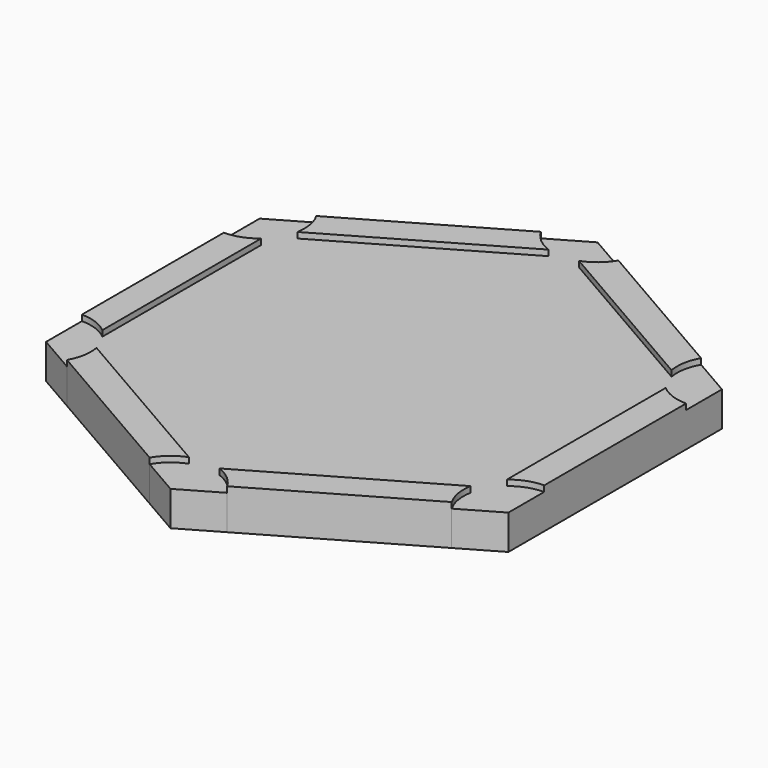
from build123d import *

# Parameters (mm, degrees)
F1_DEPTH        = 6
F2_DEPTH        = 7
F2_COPIES_COUNT = 6
F4_DEPTH        = 5
F5_START        = 1
F5_DEPTH        = 4


# Not quite as in the source:
# - a pattern or mirror of a feature is missing from the dataset's text; its kind, count and spacing are read off the source's solid


with BuildPart() as f1:
    # F0 (on Top) → F1 (new body)
    with BuildSketch(Plane.XY):
        with BuildLine():
            ThreePointArc((-33.2883031207, -26.9690107676), (-32.3656613578, -24.4279423614), (-32.3719521258, -21.7245635692))
            Line((-32.3719521258, -21.7245635692), (-35, -20.2072594216))
            Line((-35, -20.2072594216), (-35, -17.1726511264))
            ThreePointArc((-35, -17.1726511264), (-37.3380493261, -15.8155137655), (-40, -15.3440107676))
            Line((-40, -15.3440107676), (-40, -23.0940107676))
            Line((-40, -23.0940107676), (-33.2883031207, -26.9690107676))
        make_face()
        with BuildLine():
            Line((0, -46.1880215352), (6.7116968793, -42.3130215352))
            ThreePointArc((6.7116968793, -42.3130215352), (4.9723879682, -40.2434561269), (2.6280478742, -38.8972146957))
            Line((2.6280478742, -38.8972146957), (0, -40.4145188433))
            Line((0, -40.4145188433), (-2.6280478742, -38.8972146957))
            ThreePointArc((-2.6280478742, -38.8972146957), (-4.9723879682, -40.2434561269), (-6.7116968793, -42.3130215352))
            Line((-6.7116968793, -42.3130215352), (0, -46.1880215352))
        make_face()
        with BuildLine():
            Line((40, -23.0940107676), (40, -15.3440107676))
            ThreePointArc((40, -15.3440107676), (37.3380493261, -15.8155137655), (35, -17.1726511264))
            Line((35, -17.1726511264), (35, -20.2072594216))
            Line((35, -20.2072594216), (32.3719521258, -21.7245635692))
            ThreePointArc((32.3719521258, -21.7245635692), (32.3656613578, -24.4279423614), (33.2883031207, -26.9690107676))
            Line((33.2883031207, -26.9690107676), (40, -23.0940107676))
        make_face()
        with BuildLine():
            Line((40, 15.3440107676), (40, 23.0940107676))
            Line((40, 23.0940107676), (33.2883031207, 26.9690107676))
            ThreePointArc((33.2883031207, 26.9690107676), (32.3656613578, 24.4279423614), (32.3719521258, 21.7245635692))
            Line((32.3719521258, 21.7245635692), (35, 20.2072594216))
            Line((35, 20.2072594216), (35, 17.1726511264))
            ThreePointArc((35, 17.1726511264), (37.3380493261, 15.8155137655), (40, 15.3440107676))
        make_face()
        with BuildLine():
            ThreePointArc((2.6280478742, 38.8972146957), (4.9723879682, 40.2434561269), (6.7116968793, 42.3130215352))
            Line((6.7116968793, 42.3130215352), (0, 46.1880215352))
            Line((0, 46.1880215352), (-6.7116968793, 42.3130215352))
            ThreePointArc((-6.7116968793, 42.3130215352), (-4.9723879682, 40.2434561269), (-2.6280478742, 38.8972146957))
            Line((-2.6280478742, 38.8972146957), (0, 40.4145188433))
            Line((0, 40.4145188433), (2.6280478742, 38.8972146957))
        make_face()
        with BuildLine():
            ThreePointArc((-32.3719521258, 21.7245635692), (-32.3656613578, 24.4279423614), (-33.2883031207, 26.9690107676))
            Line((-33.2883031207, 26.9690107676), (-40, 23.0940107676))
            Line((-40, 23.0940107676), (-40, 15.3440107676))
            ThreePointArc((-40, 15.3440107676), (-37.3380493261, 15.8155137655), (-35, 17.1726511264))
            Line((-35, 17.1726511264), (-35, 20.2072594216))
            Line((-35, 20.2072594216), (-32.3719521258, 21.7245635692))
        make_face()
        with BuildLine():
            ThreePointArc((-35, 17.1726511264), (-33.2883031207, 19.2190107676), (-32.3719521258, 21.7245635692))
            Line((-32.3719521258, 21.7245635692), (-35, 20.2072594216))
            Line((-35, 20.2072594216), (-35, 17.1726511264))
        make_face()
        with BuildLine():
            ThreePointArc((-2.6280478742, 38.8972146957), (0, 38.4380215352), (2.6280478742, 38.8972146957))
            Line((2.6280478742, 38.8972146957), (0, 40.4145188433))
            Line((0, 40.4145188433), (-2.6280478742, 38.8972146957))
        make_face()
        with BuildLine():
            Line((-35, -20.2072594216), (-32.3719521258, -21.7245635692))
            ThreePointArc((-32.3719521258, -21.7245635692), (-33.2883031207, -19.2190107676), (-35, -17.1726511264))
            Line((-35, -17.1726511264), (-35, -20.2072594216))
        make_face()
        with BuildLine():
            Line((0, -40.4145188433), (2.6280478742, -38.8972146957))
            ThreePointArc((2.6280478742, -38.8972146957), (0, -38.4380215352), (-2.6280478742, -38.8972146957))
            Line((-2.6280478742, -38.8972146957), (0, -40.4145188433))
        make_face()
        with BuildLine():
            Line((35, -20.2072594216), (35, -17.1726511264))
            ThreePointArc((35, -17.1726511264), (33.2883031207, -19.2190107676), (32.3719521258, -21.7245635692))
            Line((32.3719521258, -21.7245635692), (35, -20.2072594216))
        make_face()
        with BuildLine():
            ThreePointArc((32.3719521258, 21.7245635692), (33.2883031207, 19.2190107676), (35, 17.1726511264))
            Line((35, 17.1726511264), (35, 20.2072594216))
            Line((35, 20.2072594216), (32.3719521258, 21.7245635692))
        make_face()
        with BuildLine():
            Line((35, -17.1726511264), (35, 17.1726511264))
            ThreePointArc((35, 17.1726511264), (33.2883031207, 19.2190107676), (32.3719521258, 21.7245635692))
            Line((32.3719521258, 21.7245635692), (2.6280478742, 38.8972146957))
            ThreePointArc((2.6280478742, 38.8972146957), (0, 38.4380215352), (-2.6280478742, 38.8972146957))
            Line((-2.6280478742, 38.8972146957), (-32.3719521258, 21.7245635692))
            ThreePointArc((-32.3719521258, 21.7245635692), (-33.2883031207, 19.2190107676), (-35, 17.1726511264))
            Line((-35, 17.1726511264), (-35, -17.1726511264))
            ThreePointArc((-35, -17.1726511264), (-33.2883031207, -19.2190107676), (-32.3719521258, -21.7245635692))
            Line((-32.3719521258, -21.7245635692), (-2.6280478742, -38.8972146957))
            ThreePointArc((-2.6280478742, -38.8972146957), (0, -38.4380215352), (2.6280478742, -38.8972146957))
            Line((2.6280478742, -38.8972146957), (32.3719521258, -21.7245635692))
            ThreePointArc((32.3719521258, -21.7245635692), (33.2883031207, -19.2190107676), (35, -17.1726511264))
        make_face()
    extrude(amount=F1_DEPTH)

    # F0 (on Top) → F2 (join)
    with BuildSketch(Plane.XY):
        with BuildLine():
            Line((40, -15.3440107676), (40, 15.3440107676))
            ThreePointArc((40, 15.3440107676), (37.3380493261, 15.8155137655), (35, 17.1726511264))
            Line((35, 17.1726511264), (35, -17.1726511264))
            ThreePointArc((35, -17.1726511264), (37.3380493261, -15.8155137655), (40, -15.3440107676))
        make_face()
    f2 = extrude(amount=F2_DEPTH)

    # F2_copies: F2 ×6 about axis
    f2_copies_axis = Axis((0, 0, 0), (0, 0, 1))
    for i in range(1, F2_COPIES_COUNT):
        add(f2.rotate(f2_copies_axis, i * 360 / F2_COPIES_COUNT))

    # F3 (on face) → F4 (cut)
    with BuildSketch(Plane.XY):
        with BuildLine():
            Line((-36, -12.1346096908), (-36, -7.4346096908))
            ThreePointArc((-36, -7.4346096908), (-38.35, -9.7846096908), (-36, -12.1346096908))
        make_face()
        with BuildLine():
            ThreePointArc((-33.65, -9.7846096908), (-34.3382990642, -8.122908755), (-36, -7.4346096908))
            Line((-36, -7.4346096908), (-36, -12.1346096908))
            ThreePointArc((-36, -12.1346096908), (-34.3382990642, -11.4463106266), (-33.65, -9.7846096908))
        make_face()
        with BuildLine():
            ThreePointArc((-33.65, 9.7846096908), (-34.3382990642, 11.4463106266), (-36, 12.1346096908))
            Line((-36, 12.1346096908), (-36, 7.4346096908))
            ThreePointArc((-36, 7.4346096908), (-34.3382990642, 8.122908755), (-33.65, 9.7846096908))
        make_face()
        with BuildLine():
            Line((-36, 7.4346096908), (-36, 12.1346096908))
            ThreePointArc((-36, 12.1346096908), (-38.35, 9.7846096908), (-36, 7.4346096908))
        make_face()
        with BuildLine():
            ThreePointArc((-24.1237205584, 26.2846096908), (-24.2037948666, 26.8928344468), (-24.4385608595, 27.4596096908))
            Line((-24.4385608595, 27.4596096908), (-28.5088802573, 25.1096096908))
            ThreePointArc((-28.5088802573, 25.1096096908), (-25.8654958024, 24.014683999), (-24.1237205584, 26.2846096908))
        make_face()
        with BuildLine():
            Line((-28.5088802573, 25.1096096908), (-24.4385608595, 27.4596096908))
            ThreePointArc((-24.4385608595, 27.4596096908), (-27.6487205584, 28.3197693897), (-28.5088802573, 25.1096096908))
        make_face()
        with BuildLine():
            ThreePointArc((-7.1762794416, 36.0692193817), (-7.2563537498, 36.6774441376), (-7.4911197427, 37.2442193817))
            Line((-7.4911197427, 37.2442193817), (-11.5614391405, 34.8942193817))
            ThreePointArc((-11.5614391405, 34.8942193817), (-8.9180546856, 33.7992936899), (-7.1762794416, 36.0692193817))
        make_face()
        with BuildLine():
            Line((-11.5614391405, 34.8942193817), (-7.4911197427, 37.2442193817))
            ThreePointArc((-7.4911197427, 37.2442193817), (-10.7012794416, 38.1043790805), (-11.5614391405, 34.8942193817))
        make_face()
        with BuildLine():
            ThreePointArc((7.4911197427, 37.2442193817), (8.3512794416, 34.0340596828), (11.5614391405, 34.8942193817))
            Line((11.5614391405, 34.8942193817), (7.4911197427, 37.2442193817))
        make_face()
        with BuildLine():
            Line((7.4911197427, 37.2442193817), (11.5614391405, 34.8942193817))
            ThreePointArc((11.5614391405, 34.8942193817), (11.7962051334, 35.4609946257), (11.8762794416, 36.0692193817))
            ThreePointArc((11.8762794416, 36.0692193817), (10.1345041976, 38.3391450734), (7.4911197427, 37.2442193817))
        make_face()
        with BuildLine():
            ThreePointArc((24.4385608595, 27.4596096908), (25.2987205584, 24.2494499919), (28.5088802573, 25.1096096908))
            Line((28.5088802573, 25.1096096908), (24.4385608595, 27.4596096908))
        make_face()
        with BuildLine():
            Line((24.4385608595, 27.4596096908), (28.5088802573, 25.1096096908))
            ThreePointArc((28.5088802573, 25.1096096908), (28.7436462502, 25.6763849348), (28.8237205584, 26.2846096908))
            ThreePointArc((28.8237205584, 26.2846096908), (27.0819453144, 28.5545353826), (24.4385608595, 27.4596096908))
        make_face()
        with BuildLine():
            Line((36, 7.4346096908), (36, 12.1346096908))
            ThreePointArc((36, 12.1346096908), (33.65, 9.7846096908), (36, 7.4346096908))
        make_face()
        with BuildLine():
            ThreePointArc((38.35, 9.7846096908), (37.6617009358, 11.4463106266), (36, 12.1346096908))
            Line((36, 12.1346096908), (36, 7.4346096908))
            ThreePointArc((36, 7.4346096908), (37.6617009358, 8.122908755), (38.35, 9.7846096908))
        make_face()
        with BuildLine():
            Line((36, -12.1346096908), (36, -7.4346096908))
            ThreePointArc((36, -7.4346096908), (33.65, -9.7846096908), (36, -12.1346096908))
        make_face()
        with BuildLine():
            ThreePointArc((38.35, -9.7846096908), (37.6617009358, -8.122908755), (36, -7.4346096908))
            Line((36, -7.4346096908), (36, -12.1346096908))
            ThreePointArc((36, -12.1346096908), (37.6617009358, -11.4463106266), (38.35, -9.7846096908))
        make_face()
        with BuildLine():
            ThreePointArc((28.8237205584, -26.2846096908), (28.7436462502, -25.6763849348), (28.5088802573, -25.1096096908))
            Line((28.5088802573, -25.1096096908), (24.4385608595, -27.4596096908))
            ThreePointArc((24.4385608595, -27.4596096908), (27.0819453144, -28.5545353826), (28.8237205584, -26.2846096908))
        make_face()
        with BuildLine():
            Line((24.4385608595, -27.4596096908), (28.5088802573, -25.1096096908))
            ThreePointArc((28.5088802573, -25.1096096908), (25.2987205584, -24.2494499919), (24.4385608595, -27.4596096908))
        make_face()
        with BuildLine():
            ThreePointArc((11.8762794416, -36.0692193817), (11.7962051334, -35.4609946257), (11.5614391405, -34.8942193817))
            Line((11.5614391405, -34.8942193817), (7.4911197427, -37.2442193817))
            ThreePointArc((7.4911197427, -37.2442193817), (10.1345041976, -38.3391450734), (11.8762794416, -36.0692193817))
        make_face()
        with BuildLine():
            Line((7.4911197427, -37.2442193817), (11.5614391405, -34.8942193817))
            ThreePointArc((11.5614391405, -34.8942193817), (8.3512794416, -34.0340596828), (7.4911197427, -37.2442193817))
        make_face()
        with BuildLine():
            Line((-9.5262794416, -36.0692193817), (-7.4911197427, -37.2442193817))
            ThreePointArc((-7.4911197427, -37.2442193817), (-7.2563537498, -36.6774441376), (-7.1762794416, -36.0692193817))
            ThreePointArc((-7.1762794416, -36.0692193817), (-8.9180546856, -33.7992936899), (-11.5614391405, -34.8942193817))
            Line((-11.5614391405, -34.8942193817), (-9.5262794416, -36.0692193817))
        make_face()
        with BuildLine():
            ThreePointArc((-11.5614391405, -34.8942193817), (-10.7012794416, -38.1043790805), (-7.4911197427, -37.2442193817))
            Line((-7.4911197427, -37.2442193817), (-9.5262794416, -36.0692193817))
            Line((-9.5262794416, -36.0692193817), (-11.5614391405, -34.8942193817))
        make_face()
        with BuildLine():
            Line((-26.4737205584, -26.2846096908), (-24.4385608595, -27.4596096908))
            ThreePointArc((-24.4385608595, -27.4596096908), (-24.2037948666, -26.8928344468), (-24.1237205584, -26.2846096908))
            ThreePointArc((-24.1237205584, -26.2846096908), (-25.8654958024, -24.014683999), (-28.5088802573, -25.1096096908))
            Line((-28.5088802573, -25.1096096908), (-26.4737205584, -26.2846096908))
        make_face()
        with BuildLine():
            ThreePointArc((-28.5088802573, -25.1096096908), (-27.6487205584, -28.3197693897), (-24.4385608595, -27.4596096908))
            Line((-24.4385608595, -27.4596096908), (-26.4737205584, -26.2846096908))
            Line((-26.4737205584, -26.2846096908), (-28.5088802573, -25.1096096908))
        make_face()
    extrude(amount=F4_DEPTH, mode=Mode.SUBTRACT)

    # F3 (on face) → F5 (cut)
    with BuildSketch(Plane.XY.offset(F5_START)):
        with BuildLine():
            ThreePointArc((39.5, 11.7211013639), (38.0315060063, 13.2303292595), (36, 13.7846096908))
            Line((36, 13.7846096908), (36, 12.1346096908))
            ThreePointArc((36, 12.1346096908), (37.6617009358, 11.4463106266), (38.35, 9.7846096908))
            ThreePointArc((38.35, 9.7846096908), (37.6617009358, 8.122908755), (36, 7.4346096908))
            Line((36, 7.4346096908), (36, 5.7846096908))
            ThreePointArc((36, 5.7846096908), (38.0315060063, 6.3388901221), (39.5, 7.8481180177))
            Line((39.5, 7.8481180177), (39.5, 11.7211013639))
        make_face()
        with BuildLine():
            Line((36, 12.1346096908), (36, 13.7846096908))
            ThreePointArc((36, 13.7846096908), (32, 9.7846096908), (36, 5.7846096908))
            Line((36, 5.7846096908), (36, 7.4346096908))
            ThreePointArc((36, 7.4346096908), (33.65, 9.7846096908), (36, 12.1346096908))
        make_face()
        with BuildLine():
            ThreePointArc((23.0096189432, 28.2846096908), (24.4737205584, 22.8205080757), (29.9378221735, 24.2846096908))
            Line((29.9378221735, 24.2846096908), (28.5088802573, 25.1096096908))
            ThreePointArc((28.5088802573, 25.1096096908), (25.2987205584, 24.2494499919), (24.4385608595, 27.4596096908))
            Line((24.4385608595, 27.4596096908), (23.0096189432, 28.2846096908))
        make_face()
        with BuildLine():
            Line((28.5088802573, 25.1096096908), (29.9378221735, 24.2846096908))
            ThreePointArc((29.9378221735, 24.2846096908), (30.4735542424, 26.3210857159), (29.9007715415, 28.3474527675))
            Line((29.9007715415, 28.3474527675), (26.5466695752, 30.2839444406))
            ThreePointArc((26.5466695752, 30.2839444406), (24.5053928807, 29.7668052846), (23.0096189432, 28.2846096908))
            Line((23.0096189432, 28.2846096908), (24.4385608595, 27.4596096908))
            ThreePointArc((24.4385608595, 27.4596096908), (27.0819453144, 28.5545353826), (28.8237205584, 26.2846096908))
            ThreePointArc((28.8237205584, 26.2846096908), (28.7436462502, 25.6763849348), (28.5088802573, 25.1096096908))
        make_face()
        with BuildLine():
            ThreePointArc((39.5, -7.8481180177), (38.0315060063, -6.3388901221), (36, -5.7846096908))
            Line((36, -5.7846096908), (36, -7.4346096908))
            ThreePointArc((36, -7.4346096908), (37.6617009358, -8.122908755), (38.35, -9.7846096908))
            ThreePointArc((38.35, -9.7846096908), (37.6617009358, -11.4463106266), (36, -12.1346096908))
            Line((36, -12.1346096908), (36, -13.7846096908))
            ThreePointArc((36, -13.7846096908), (38.0315060063, -13.2303292595), (39.5, -11.7211013639))
            Line((39.5, -11.7211013639), (39.5, -7.8481180177))
        make_face()
        with BuildLine():
            Line((36, -7.4346096908), (36, -5.7846096908))
            ThreePointArc((36, -5.7846096908), (32, -9.7846096908), (36, -13.7846096908))
            Line((36, -13.7846096908), (36, -12.1346096908))
            ThreePointArc((36, -12.1346096908), (33.65, -9.7846096908), (36, -7.4346096908))
        make_face()
        with BuildLine():
            ThreePointArc((6.0621778265, 38.0692193817), (7.5262794416, 32.6051177665), (12.9903810568, 34.0692193817))
            Line((12.9903810568, 34.0692193817), (11.5614391405, 34.8942193817))
            ThreePointArc((11.5614391405, 34.8942193817), (8.3512794416, 34.0340596828), (7.4911197427, 37.2442193817))
            Line((7.4911197427, 37.2442193817), (6.0621778265, 38.0692193817))
        make_face()
        with BuildLine():
            Line((11.5614391405, 34.8942193817), (12.9903810568, 34.0692193817))
            ThreePointArc((12.9903810568, 34.0692193817), (13.5261131256, 36.1056954067), (12.9533304248, 38.1320624583))
            Line((12.9533304248, 38.1320624583), (9.5992284585, 40.0685541315))
            ThreePointArc((9.5992284585, 40.0685541315), (7.557951764, 39.5514149754), (6.0621778265, 38.0692193817))
            Line((6.0621778265, 38.0692193817), (7.4911197427, 37.2442193817))
            ThreePointArc((7.4911197427, 37.2442193817), (10.1345041976, 38.3391450734), (11.8762794416, 36.0692193817))
            ThreePointArc((11.8762794416, 36.0692193817), (11.7962051334, 35.4609946257), (11.5614391405, 34.8942193817))
        make_face()
        with BuildLine():
            ThreePointArc((29.9007715415, -28.3474527675), (30.4735542424, -26.3210857159), (29.9378221735, -24.2846096908))
            Line((29.9378221735, -24.2846096908), (28.5088802573, -25.1096096908))
            ThreePointArc((28.5088802573, -25.1096096908), (28.7436462502, -25.6763849348), (28.8237205584, -26.2846096908))
            ThreePointArc((28.8237205584, -26.2846096908), (27.0819453144, -28.5545353826), (24.4385608595, -27.4596096908))
            Line((24.4385608595, -27.4596096908), (23.0096189432, -28.2846096908))
            ThreePointArc((23.0096189432, -28.2846096908), (24.5053928807, -29.7668052846), (26.5466695752, -30.2839444406))
            Line((26.5466695752, -30.2839444406), (29.9007715415, -28.3474527675))
        make_face()
        with BuildLine():
            Line((28.5088802573, -25.1096096908), (29.9378221735, -24.2846096908))
            ThreePointArc((29.9378221735, -24.2846096908), (24.4737205584, -22.8205080757), (23.0096189432, -28.2846096908))
            Line((23.0096189432, -28.2846096908), (24.4385608595, -27.4596096908))
            ThreePointArc((24.4385608595, -27.4596096908), (25.2987205584, -24.2494499919), (28.5088802573, -25.1096096908))
        make_face()
        with BuildLine():
            ThreePointArc((-12.9903810568, 34.0692193817), (-7.5262794416, 32.6051177665), (-6.0621778265, 38.0692193817))
            Line((-6.0621778265, 38.0692193817), (-7.4911197427, 37.2442193817))
            ThreePointArc((-7.4911197427, 37.2442193817), (-7.2563537498, 36.6774441376), (-7.1762794416, 36.0692193817))
            ThreePointArc((-7.1762794416, 36.0692193817), (-8.9180546856, 33.7992936899), (-11.5614391405, 34.8942193817))
            Line((-11.5614391405, 34.8942193817), (-12.9903810568, 34.0692193817))
        make_face()
        with BuildLine():
            Line((-7.4911197427, 37.2442193817), (-6.0621778265, 38.0692193817))
            ThreePointArc((-6.0621778265, 38.0692193817), (-7.557951764, 39.5514149754), (-9.5992284585, 40.0685541315))
            Line((-9.5992284585, 40.0685541315), (-12.9533304248, 38.1320624583))
            ThreePointArc((-12.9533304248, 38.1320624583), (-13.5261131256, 36.1056954067), (-12.9903810568, 34.0692193817))
            Line((-12.9903810568, 34.0692193817), (-11.5614391405, 34.8942193817))
            ThreePointArc((-11.5614391405, 34.8942193817), (-10.7012794416, 38.1043790805), (-7.4911197427, 37.2442193817))
        make_face()
        with BuildLine():
            ThreePointArc((12.9533304248, -38.1320624583), (13.5261131256, -36.1056954067), (12.9903810568, -34.0692193817))
            Line((12.9903810568, -34.0692193817), (11.5614391405, -34.8942193817))
            ThreePointArc((11.5614391405, -34.8942193817), (11.7962051334, -35.4609946257), (11.8762794416, -36.0692193817))
            ThreePointArc((11.8762794416, -36.0692193817), (10.1345041976, -38.3391450734), (7.4911197427, -37.2442193817))
            Line((7.4911197427, -37.2442193817), (6.0621778265, -38.0692193817))
            ThreePointArc((6.0621778265, -38.0692193817), (7.557951764, -39.5514149754), (9.5992284585, -40.0685541315))
            Line((9.5992284585, -40.0685541315), (12.9533304248, -38.1320624583))
        make_face()
        with BuildLine():
            Line((11.5614391405, -34.8942193817), (12.9903810568, -34.0692193817))
            ThreePointArc((12.9903810568, -34.0692193817), (7.5262794416, -32.6051177665), (6.0621778265, -38.0692193817))
            Line((6.0621778265, -38.0692193817), (7.4911197427, -37.2442193817))
            ThreePointArc((7.4911197427, -37.2442193817), (8.3512794416, -34.0340596828), (11.5614391405, -34.8942193817))
        make_face()
        with BuildLine():
            ThreePointArc((-29.9378221735, 24.2846096908), (-24.4737205584, 22.8205080757), (-23.0096189432, 28.2846096908))
            Line((-23.0096189432, 28.2846096908), (-24.4385608595, 27.4596096908))
            ThreePointArc((-24.4385608595, 27.4596096908), (-24.2037948666, 26.8928344468), (-24.1237205584, 26.2846096908))
            ThreePointArc((-24.1237205584, 26.2846096908), (-25.8654958024, 24.014683999), (-28.5088802573, 25.1096096908))
            Line((-28.5088802573, 25.1096096908), (-29.9378221735, 24.2846096908))
        make_face()
        with BuildLine():
            Line((-24.4385608595, 27.4596096908), (-23.0096189432, 28.2846096908))
            ThreePointArc((-23.0096189432, 28.2846096908), (-24.5053928807, 29.7668052846), (-26.5466695752, 30.2839444406))
            Line((-26.5466695752, 30.2839444406), (-29.9007715415, 28.3474527675))
            ThreePointArc((-29.9007715415, 28.3474527675), (-30.4735542424, 26.3210857159), (-29.9378221735, 24.2846096908))
            Line((-29.9378221735, 24.2846096908), (-28.5088802573, 25.1096096908))
            ThreePointArc((-28.5088802573, 25.1096096908), (-27.6487205584, 28.3197693897), (-24.4385608595, 27.4596096908))
        make_face()
        with BuildLine():
            ThreePointArc((-9.5992284585, -40.0685541315), (-7.557951764, -39.5514149754), (-6.0621778265, -38.0692193817))
            Line((-6.0621778265, -38.0692193817), (-7.4911197427, -37.2442193817))
            ThreePointArc((-7.4911197427, -37.2442193817), (-10.7012794416, -38.1043790805), (-11.5614391405, -34.8942193817))
            Line((-11.5614391405, -34.8942193817), (-12.9903810568, -34.0692193817))
            ThreePointArc((-12.9903810568, -34.0692193817), (-13.5261131256, -36.1056954067), (-12.9533304248, -38.1320624583))
            Line((-12.9533304248, -38.1320624583), (-9.5992284585, -40.0685541315))
        make_face()
        with BuildLine():
            Line((-7.4911197427, -37.2442193817), (-6.0621778265, -38.0692193817))
            ThreePointArc((-6.0621778265, -38.0692193817), (-7.5262794416, -32.6051177665), (-12.9903810568, -34.0692193817))
            Line((-12.9903810568, -34.0692193817), (-11.5614391405, -34.8942193817))
            ThreePointArc((-11.5614391405, -34.8942193817), (-8.9180546856, -33.7992936899), (-7.1762794416, -36.0692193817))
            ThreePointArc((-7.1762794416, -36.0692193817), (-7.2563537498, -36.6774441376), (-7.4911197427, -37.2442193817))
        make_face()
        with BuildLine():
            ThreePointArc((-36, 5.7846096908), (-32, 9.7846096908), (-36, 13.7846096908))
            Line((-36, 13.7846096908), (-36, 12.1346096908))
            ThreePointArc((-36, 12.1346096908), (-34.3382990642, 11.4463106266), (-33.65, 9.7846096908))
            ThreePointArc((-33.65, 9.7846096908), (-34.3382990642, 8.122908755), (-36, 7.4346096908))
            Line((-36, 7.4346096908), (-36, 5.7846096908))
        make_face()
        with BuildLine():
            Line((-36, 12.1346096908), (-36, 13.7846096908))
            ThreePointArc((-36, 13.7846096908), (-38.0315060063, 13.2303292595), (-39.5, 11.7211013639))
            Line((-39.5, 11.7211013639), (-39.5, 7.8481180177))
            ThreePointArc((-39.5, 7.8481180177), (-38.0315060063, 6.3388901221), (-36, 5.7846096908))
            Line((-36, 5.7846096908), (-36, 7.4346096908))
            ThreePointArc((-36, 7.4346096908), (-38.35, 9.7846096908), (-36, 12.1346096908))
        make_face()
        with BuildLine():
            ThreePointArc((-26.5466695752, -30.2839444406), (-24.5053928807, -29.7668052846), (-23.0096189432, -28.2846096908))
            Line((-23.0096189432, -28.2846096908), (-24.4385608595, -27.4596096908))
            ThreePointArc((-24.4385608595, -27.4596096908), (-27.6487205584, -28.3197693897), (-28.5088802573, -25.1096096908))
            Line((-28.5088802573, -25.1096096908), (-29.9378221735, -24.2846096908))
            ThreePointArc((-29.9378221735, -24.2846096908), (-30.4735542424, -26.3210857159), (-29.9007715415, -28.3474527675))
            Line((-29.9007715415, -28.3474527675), (-26.5466695752, -30.2839444406))
        make_face()
        with BuildLine():
            Line((-24.4385608595, -27.4596096908), (-23.0096189432, -28.2846096908))
            ThreePointArc((-23.0096189432, -28.2846096908), (-24.4737205584, -22.8205080757), (-29.9378221735, -24.2846096908))
            Line((-29.9378221735, -24.2846096908), (-28.5088802573, -25.1096096908))
            ThreePointArc((-28.5088802573, -25.1096096908), (-25.8654958024, -24.014683999), (-24.1237205584, -26.2846096908))
            ThreePointArc((-24.1237205584, -26.2846096908), (-24.2037948666, -26.8928344468), (-24.4385608595, -27.4596096908))
        make_face()
        with BuildLine():
            ThreePointArc((-36, -13.7846096908), (-32, -9.7846096908), (-36, -5.7846096908))
            Line((-36, -5.7846096908), (-36, -7.4346096908))
            ThreePointArc((-36, -7.4346096908), (-34.3382990642, -8.122908755), (-33.65, -9.7846096908))
            ThreePointArc((-33.65, -9.7846096908), (-34.3382990642, -11.4463106266), (-36, -12.1346096908))
            Line((-36, -12.1346096908), (-36, -13.7846096908))
        make_face()
        with BuildLine():
            Line((-36, -7.4346096908), (-36, -5.7846096908))
            ThreePointArc((-36, -5.7846096908), (-38.0315060063, -6.3388901221), (-39.5, -7.8481180177))
            Line((-39.5, -7.8481180177), (-39.5, -11.7211013639))
            ThreePointArc((-39.5, -11.7211013639), (-38.0315060063, -13.2303292595), (-36, -13.7846096908))
            Line((-36, -13.7846096908), (-36, -12.1346096908))
            ThreePointArc((-36, -12.1346096908), (-38.35, -9.7846096908), (-36, -7.4346096908))
        make_face()
    extrude(amount=F5_DEPTH, mode=Mode.SUBTRACT)


solid = f1.part
